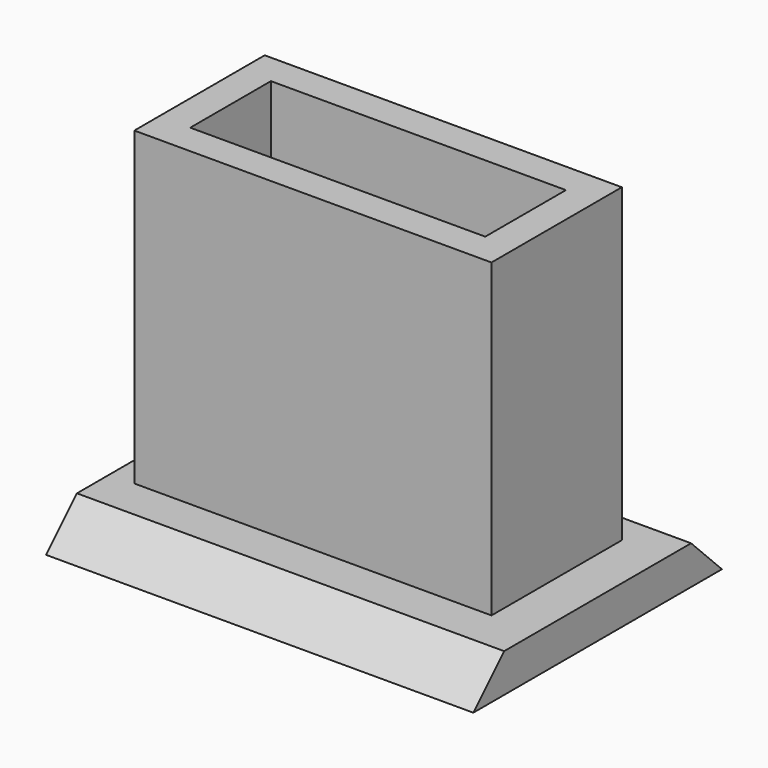
from build123d import *

# Parameters (mm, degrees)
F0_W        = 34.925
F0_H        = 25.4
F1_DEPTH    = 3.1496
F2_SIZE     = 3.14959
F3_W        = 29.1948509403
F3_H        = 13.3209023625
F4_DEPTH    = 25.4
F5_T        = 2.54
F5_T3_DEPTH = 34.2748509403
F5_T5_DEPTH = 18.4009023625


# Not quite as in the source:
# - a fillet or chamfer is up to 0.001 mm smaller than in the source, because OpenCascade refuses the exact size
# - a shell that OpenCascade refuses in one call is made with other operations: the cavity is built on its own and cut out


with BuildPart() as f1:
    # F0 (on Top) → F1 (new body)
    with BuildSketch(Plane.XY):
        with Locations((9.7498925388, -19.8326882303)):
            Rectangle(F0_W, F0_H)
    extrude(amount=F1_DEPTH)

    # F2 (size 3.1496 in the source; OpenCascade refuses exactly that, so slightly less here)
    f2_edges = [f1.edges().sort_by_distance(p)[0] for p in [
        (9.749893, -32.532688, 3.1496),
        (9.749893, -7.132688, 3.1496),
    ]]
    chamfer(f2_edges, length=F2_SIZE)

    # F3 (on face) → F4 (join)
    with BuildSketch(Plane.XY.offset(3.1496)):
        with Locations((8.8992563542, -19.3738183007)):
            Rectangle(F3_W, F3_H)
    extrude(amount=F4_DEPTH)

    # F5: shell of thickness 2.54, made by hand


with BuildPart() as f5_core1:
    # F5_t2: copy of F1
    add(f1.part)

    # the walls: a layer under each face that stays
    f5_faces = [f5_core1.faces().sort_by_distance(p)[0] for p in [
        (27.2123925388, -19.8326882303, 1.5748),
        (9.7498925388, -32.5326882303, 5e-06),
        (9.7498925388, -30.9578932303, 1.574805),
        (9.7498925388, -19.8326882303, 0),
        (-1.8917741279, -26.1996282303, 3.1496),
        (9.7498925388, -7.1326882303, 5e-06),
        (9.7498925388, -8.7074832303, 1.574805),
        (-7.7126074612, -19.8326882303, 1.5748),
        (8.8992563542, -12.7133671194, 15.8496),
        (-5.6981691159, -19.3738183007, 15.8496),
        (8.8992563542, -26.0342694819, 15.8496),
        (23.4966818243, -19.3738183007, 15.8496),
    ]]
    thicken(f5_faces, amount=-F5_T, mode=Mode.SUBTRACT)

    # F5_s4 → F5_t3 (cut)
    with BuildSketch(Plane.YZ.offset(-8.2381691159)):
        Polygon((-12.6879671194, 3.175), (-12.7133671194, 0.6096), (-15.2533671194, 0.6096), (-15.2533671194, 3.1496), align=None)
        Polygon((-26.0596694819, 3.175), (-26.0342694819, 0.6096), (-23.4942694819, 0.6096), (-23.4942694819, 3.1496), align=None)
    extrude(amount=F5_T3_DEPTH, mode=Mode.SUBTRACT)

    # F5_s6 → F5_t5 (cut)
    with BuildSketch(Plane.XZ.offset(10.1733671194)):
        Polygon((-5.7235691159, 3.175), (-5.6981691159, 0.6096), (-3.1581691159, 0.6096), (-3.1581691159, 3.1496), align=None)
        Polygon((23.5220818243, 3.175), (23.4966818243, 0.6096), (20.9566818243, 0.6096), (20.9566818243, 3.1496), align=None)
    extrude(amount=F5_T5_DEPTH, mode=Mode.SUBTRACT)


with BuildPart() as f1_1:
    add(f1.part)

    # what is left inside the walls is the cavity
    f5_cavity = [f5_core1.part.solids().sort_by_distance(p)[0] for p in [
        (12.918398, -15.278767, 15.5448),
    ]]
    add(f5_cavity, mode=Mode.SUBTRACT)


solid = f1_1.part
